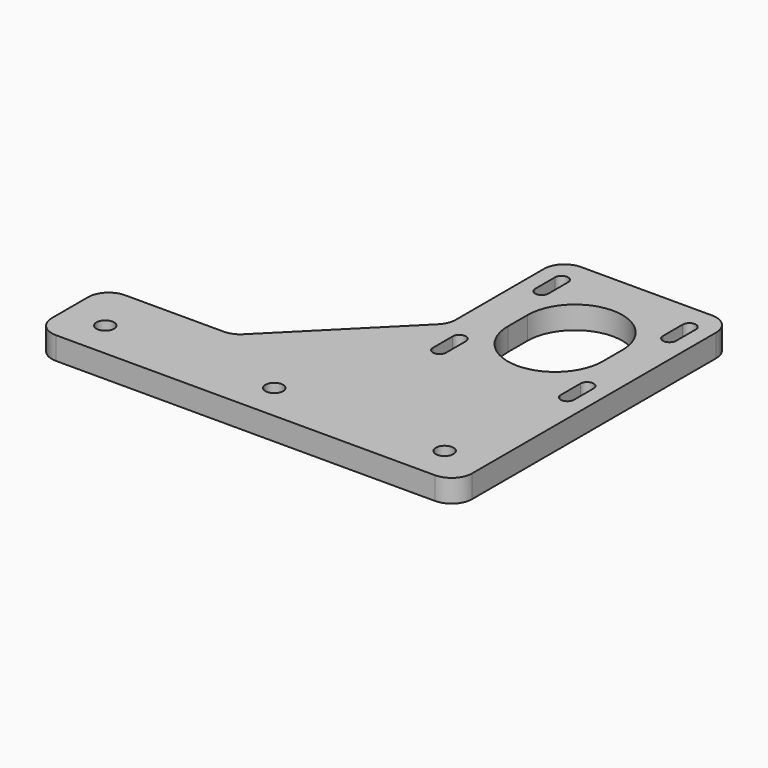
from build123d import *

# Parameters (mm, degrees)
F0_R     = 2.13
F1_DEPTH = 5.5


# Not quite as in the source:
# - ends of sketch curves that miss each other by under 0.0002 mm in the source are joined


with BuildPart() as f1:
    # F0 (on Top) → F1 (new body)
    with BuildSketch(Plane.XY):
        with BuildLine():
            ThreePointArc((9.1999998704, 10.271), (8.8197324019, 8.3578320272), (7.735999997, 6.736000003))
            Line((7.735999997, 6.736000003), (-18.536, -19.536))
            ThreePointArc((-18.536, -19.536), (-20.1578320272, -20.6197324019), (-22.071, -20.9999998704))
            Line((-22.071, -20.9999998704), (-46, -21))
            ThreePointArc((-46, -21), (-49.5349996687, -22.4650003313), (-50.9999996674, -26.0000000001))
            Line((-50.9999996674, -26.0000000001), (-51, -37))
            ThreePointArc((-51, -37), (-49.5349996687, -40.5349996687), (-45.9999999999, -41.9999996674))
            Line((-45.9999999999, -41.9999996674), (46, -42))
            ThreePointArc((46, -42), (49.5349996687, -40.5349996687), (50.9999996674, -36.9999999999))
            Line((50.9999996674, -36.9999999999), (51, 37))
            ThreePointArc((51, 37), (49.5349996687, 40.5349996687), (45.9999999999, 41.9999996674))
            Line((45.9999999999, 41.9999996674), (14.2, 42))
            ThreePointArc((14.2, 42), (10.6650003313, 40.5349996687), (9.2000003326, 36.9999999999))
            Line((9.2000003326, 36.9999999999), (9.1999998704, 10.271))
        make_face()
        with Locations((-41.17, -33.07)):
            Circle(F0_R, mode=Mode.SUBTRACT)
        with Locations((-0.17, -33.07)):
            Circle(F0_R, mode=Mode.SUBTRACT)
        with Locations((41.17, -33.07)):
            Circle(F0_R, mode=Mode.SUBTRACT)
        with BuildLine():
            ThreePointArc((13, 4.6), (14.6, 6.2), (16.2, 4.6))
            Line((16.2, 4.6), (16.2, -1.4))
            ThreePointArc((16.2, -1.4), (14.6, -3), (13, -1.4))
            Line((13, -1.4), (13, 4.6))
        make_face(mode=Mode.SUBTRACT)
        with BuildLine():
            Line((47.2, 4.6), (47.2, -1.4))
            ThreePointArc((47.2, -1.4), (45.6, -3), (44, -1.4))
            Line((44, -1.4), (44, 4.6))
            ThreePointArc((44, 4.6), (45.6, 6.2), (47.2, 4.6))
        make_face(mode=Mode.SUBTRACT)
        with BuildLine():
            ThreePointArc((41.6, 14.3), (30.1, 2.8), (18.6, 14.3))
            Line((18.6, 14.3), (18.6, 20.3))
            ThreePointArc((18.6, 20.3), (30.1, 31.8), (41.6, 20.3))
            Line((41.6, 20.3), (41.6, 14.3))
        make_face(mode=Mode.SUBTRACT)
        with BuildLine():
            ThreePointArc((13, 35.6), (14.6, 37.2), (16.2, 35.6))
            Line((16.2, 35.6), (16.2, 29.6))
            ThreePointArc((16.2, 29.6), (14.6, 28), (13, 29.6))
            Line((13, 29.6), (13, 35.6))
        make_face(mode=Mode.SUBTRACT)
        with BuildLine():
            Line((47.2, 35.6), (47.2, 29.6))
            ThreePointArc((47.2, 29.6), (45.6, 28), (44, 29.6))
            Line((44, 29.6), (44, 35.6))
            ThreePointArc((44, 35.6), (45.6, 37.2), (47.2, 35.6))
        make_face(mode=Mode.SUBTRACT)
    extrude(amount=F1_DEPTH)


solid = f1.part
